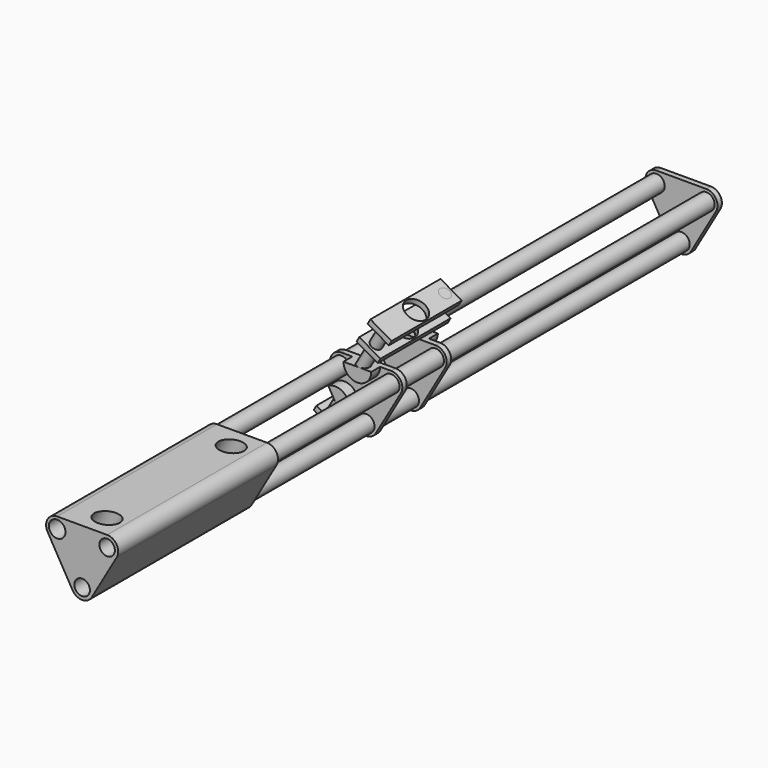
from build123d import *

# Parameters (mm, degrees)
F0_R      = 7.5
F0_R_2    = 7
F1_DEPTH  = 500
F3_DEPTH  = 5
F4_R      = 7.5
F5_DEPTH  = 180
F8_R      = 7
F9_DEPTH  = 25
F11_R     = 7
F12_DEPTH = 195.3
F15_DEPTH = 5
F18_DEPTH = 5
F20_DEPTH = 10
F22_DEPTH = 10
F24_R     = 5
F25_DEPTH = 50
F27_R     = 5
F28_DEPTH = 50
F29_W     = 22
F29_H     = 79
F30_DEPTH = 5
F31_R     = 10
F32_DEPTH = 28.9
F34_W     = 22
F34_H     = 79
F35_DEPTH = 5
F36_R     = 10
F37_DEPTH = 14.6
F39_DEPTH = 10
F41_DEPTH = 10
F44_R     = 5
F45_DEPTH = 25
F46_R     = 5
F47_DEPTH = 25.1
F48_W     = 22
F48_H     = 79
F48_R     = 5
F49_DEPTH = 5
F50_R     = 10
F51_DEPTH = 25
F52_R     = 5
F53_DEPTH = 25
F7_R      = 10
F56_DEPTH = 101


# Not quite as in the source:
# - a feature of the source that left no trace in its solid (it failed there, or was rolled back) is left out


with BuildPart() as f1:
    # F0 (on Front) → F1 (new body)
    with BuildSketch(Plane.XZ):
        with Locations((-22.5, 38.9711431703)):
            Circle(F0_R)
        with Locations((-22.5, 38.9711431703)):
            Circle(F0_R_2, mode=Mode.SUBTRACT)
    extrude(amount=F1_DEPTH)


with BuildPart() as f1b:
    # F0 (on Front) → F1, piece 2 (new body)
    with BuildSketch(Plane.XZ):
        with Locations((22.5, 38.9711431703)):
            Circle(F0_R)
        with Locations((22.5, 38.9711431703)):
            Circle(F0_R_2, mode=Mode.SUBTRACT)
    extrude(amount=F1_DEPTH)


with BuildPart() as f1c:
    # F0 (on Front) → F1, piece 3 (new body)
    with BuildSketch(Plane.XZ):
        Circle(F0_R)
        Circle(F0_R_2, mode=Mode.SUBTRACT)
    extrude(amount=F1_DEPTH)


with BuildPart() as f3:
    # F2 (on Front) → F3 (new body)
    with BuildSketch(Plane.XZ):
        with BuildLine():
            ThreePointArc((31.1602540378, 33.9711431703), (31.1602540378, 43.9711431703), (22.5, 48.9711431703))
            Line((22.5, 48.9711431703), (-22.5, 48.9711431703))
            ThreePointArc((-22.5, 48.9711431703), (-31.1602540378, 43.9711431703), (-31.1602540378, 33.9711431703))
            Line((-31.1602540378, 33.9711431703), (-8.6602540378, -5))
            ThreePointArc((-8.6602540378, -5), (0, -10), (8.6602540378, -5))
            Line((8.6602540378, -5), (31.1602540378, 33.9711431703))
        make_face()
    extrude(amount=F3_DEPTH)

    # F8 (on face) → F9 (cut)
    with BuildSketch(Plane(origin=(0, 0, 0), x_dir=(-1, 0, 0), z_dir=(0, 1, 0))):
        with Locations((-22.5, 38.9711431703)):
            Circle(F8_R)
        with Locations((22.5, 38.9711431703)):
            Circle(F8_R)
        Circle(F8_R)
    extrude(amount=-F9_DEPTH, mode=Mode.SUBTRACT)


with BuildPart() as f5:
    # F4 (on face) → F5 (new body)
    with BuildSketch(Plane.XZ.offset(500)):
        with BuildLine():
            Line((22.5, 48.9711431703), (-22.5, 48.9711431703))
            ThreePointArc((-22.5, 48.9711431703), (-31.1602540378, 43.9711431703), (-31.1602540378, 33.9711431703))
            Line((-31.1602540378, 33.9711431703), (-8.6602540378, -5))
            ThreePointArc((-8.6602540378, -5), (0, -10), (8.6602540378, -5))
            Line((8.6602540378, -5), (31.1602540378, 33.9711431703))
            ThreePointArc((31.1602540378, 33.9711431703), (31.1602540378, 43.9711431703), (22.5, 48.9711431703))
        make_face()
        with Locations((-22.5, 38.9711431703)):
            Circle(F4_R, mode=Mode.SUBTRACT)
    extrude(amount=F5_DEPTH)

    # F11 (on face) → F12 (cut)
    with BuildSketch(Plane.XZ.offset(680)):
        with Locations((22.5, 38.9711431703)):
            Circle(F11_R)
        Circle(F11_R)
        with Locations((-22.5, 38.9711431703)):
            Circle(F11_R)
    extrude(amount=-F12_DEPTH, mode=Mode.SUBTRACT)

    # F7 (on face) → F56 (cut)
    with BuildSketch(Plane(origin=(-4.3301270189, 0, -7.5), x_dir=(0.8660254038, 0, -0.5), z_dir=(0.5, 0, 0.8660254038))):
        with Locations((-18.9711431703, -660)):
            Circle(F7_R)
        with Locations((-18.9711431703, -520)):
            Circle(F7_R)
    extrude(amount=F56_DEPTH, mode=Mode.SUBTRACT)


with BuildPart() as f15:
    # F14 (on offset) → F15 (new body)
    with BuildSketch(Plane.XZ.offset(305)):
        with BuildLine():
            ThreePointArc((31.1602540378, 33.9711431703), (31.1602540378, 43.9711431703), (22.5, 48.9711431703))
            Line((22.5, 48.9711431703), (-22.5, 48.9711431703))
            ThreePointArc((-22.5, 48.9711431703), (-31.1602540378, 43.9711431703), (-31.1602540378, 33.9711431703))
            Line((-31.1602540378, 33.9711431703), (-8.6602540378, -5))
            ThreePointArc((-8.6602540378, -5), (0, -10), (8.6602540378, -5))
            Line((8.6602540378, -5), (31.1602540378, 33.9711431703))
        make_face()
    extrude(amount=F15_DEPTH)

    # F19 (on face) → F20 (join)
    with BuildSketch(Plane(origin=(0, -305, 0), x_dir=(-1, 0, 0), z_dir=(0, 1, 0))):
        with BuildLine():
            ThreePointArc((-12.5, 48.9711431703), (0, 36.4711431703), (12.5, 48.9711431703))
            Line((12.5, 48.9711431703), (-12.5, 48.9711431703))
        make_face()
    extrude(amount=F20_DEPTH)

    # F24 (on face) → F25 (join)
    with BuildSketch(Plane(origin=(18.0801270189, 0, 31.3156986041), x_dir=(0.8660254038, 0, -0.5), z_dir=(-0.5, 0, -0.8660254038))):
        with Locations((-23.3108891325, 300)):
            Circle(F24_R)
    extrude(amount=-F25_DEPTH)

    # F38 (on face) → F39 (join)
    with BuildSketch(Plane(origin=(0, -305, 0), x_dir=(-1, 0, 0), z_dir=(0, 1, 0))):
        with BuildLine():
            Line((13.6602540378, 3.6602540378), (26.1602540378, 25.3108891325))
            ThreePointArc((26.1602540378, 25.3108891325), (9.0849364905, 20.7355715851), (13.6602540378, 3.6602540378))
        make_face()
    extrude(amount=F39_DEPTH)

    # F44 (on face) → F45 (join)
    with BuildSketch(Plane(origin=(4.4198729811, 0, 7.6554445662), x_dir=(0.8660254038, 0, -0.5), z_dir=(-0.5, 0, -0.8660254038))):
        with Locations((-23.3108891325, 300)):
            Circle(F44_R)
    extrude(amount=F45_DEPTH)


with BuildPart() as f18:
    # F17 (on offset) → F18 (new body)
    with BuildSketch(Plane.XZ.offset(355)):
        with BuildLine():
            ThreePointArc((31.1602540378, 33.9711431703), (31.1602540378, 43.9711431703), (22.5, 48.9711431703))
            Line((22.5, 48.9711431703), (-22.5, 48.9711431703))
            ThreePointArc((-22.5, 48.9711431703), (-31.1602540378, 43.9711431703), (-31.1602540378, 33.9711431703))
            Line((-31.1602540378, 33.9711431703), (-8.6602540378, -5))
            ThreePointArc((-8.6602540378, -5), (0, -10), (8.6602540378, -5))
            Line((8.6602540378, -5), (31.1602540378, 33.9711431703))
        make_face()
    extrude(amount=F18_DEPTH)

    # F21 (on face) → F22 (join)
    with BuildSketch(Plane.XZ.offset(360)):
        with BuildLine():
            Line((12.5, 48.9711431703), (-12.5, 48.9711431703))
            ThreePointArc((-12.5, 48.9711431703), (0, 36.4711431703), (12.5, 48.9711431703))
        make_face()
    extrude(amount=F22_DEPTH)

    # F27 (on face) → F28 (join)
    with BuildSketch(Plane(origin=(18.0801270189, 0, 31.3156986041), x_dir=(0.8660254038, 0, -0.5), z_dir=(0.5, 0, 0.8660254038))):
        with Locations((-23.3108891325, -365)):
            Circle(F27_R)
    extrude(amount=F28_DEPTH)

    # F40 (on face) → F41 (join)
    with BuildSketch(Plane.XZ.offset(360)):
        with BuildLine():
            ThreePointArc((-13.6602540378, 3.6602540378), (-9.0849364905, 20.7355715851), (-26.1602540378, 25.3108891325))
            Line((-26.1602540378, 25.3108891325), (-13.6602540378, 3.6602540378))
        make_face()
    extrude(amount=F41_DEPTH)

    # F46 (on face) → F47 (join)
    with BuildSketch(Plane(origin=(4.4198729811, 0, 7.6554445662), x_dir=(0.8660254038, 0, -0.5), z_dir=(0.5, 0, 0.8660254038))):
        with Locations((-23.3108891325, -365)):
            Circle(F46_R)
    extrude(amount=-F47_DEPTH)

    # F48 (on face) → F49 (join)
    with BuildSketch(Plane(origin=(-8.0801270189, 0, -13.9951905284), x_dir=(0.8660254038, 0, -0.5), z_dir=(-0.5, 0, -0.8660254038))):
        with Locations((-23.3108891325, 332.5)):
            Rectangle(F48_W, F48_H)
        with Locations((-23.3108891325, 300)):
            Circle(F48_R, mode=Mode.SUBTRACT)
    extrude(amount=-F49_DEPTH)

    # F50 (on face) → F51 (cut)
    with BuildSketch(Plane(origin=(-8.0801270189, 0, -13.9951905284), x_dir=(0.8660254038, 0, -0.5), z_dir=(-0.5, 0, -0.8660254038))):
        with Locations((-23.3108891325, 332.5)):
            Circle(F50_R)
    extrude(amount=-F51_DEPTH, mode=Mode.SUBTRACT)


with BuildPart() as f30:
    # F29 (on face) → F30 (new body)
    with BuildSketch(Plane(origin=(43.0801270189, 0, 74.6169687933), x_dir=(0.8660254038, 0, -0.5), z_dir=(0.5, 0, 0.8660254038))):
        with Locations((-23.3108891325, -332.5)):
            Rectangle(F29_W, F29_H)
    extrude(amount=-F30_DEPTH)

    # F31 (on face) → F32 (cut)
    with BuildSketch(Plane(origin=(43.0801270189, 0, 74.6169687933), x_dir=(0.8660254038, 0, -0.5), z_dir=(0.5, 0, 0.8660254038))):
        with Locations((-23.3108891325, -332.5)):
            Circle(F31_R)
    extrude(amount=-F32_DEPTH, mode=Mode.SUBTRACT)


with BuildPart() as f35:
    # F34 (on offset) → F35 (new body)
    with BuildSketch(Plane(origin=(33.0801270189, 0, 57.2964607176), x_dir=(0.8660254038, 0, -0.5), z_dir=(-0.5, 0, -0.8660254038))):
        with Locations((-23.3108891325, 332.5)):
            Rectangle(F34_W, F34_H)
    extrude(amount=F35_DEPTH)

    # F36 (on face) → F37 (cut)
    with BuildSketch(Plane(origin=(33.0801270189, 0, 57.2964607176), x_dir=(0.8660254038, 0, -0.5), z_dir=(0.5, 0, 0.8660254038))):
        with Locations((-23.3108891325, -332.5)):
            Circle(F36_R)
    extrude(amount=-F37_DEPTH, mode=Mode.SUBTRACT)


with BuildPart() as f53_tool:
    # F52 (on face) → F53 (new body)
    with BuildSketch(Plane(origin=(43.0801270189, 0, 74.6169687933), x_dir=(0.8660254038, 0, -0.5), z_dir=(0.5, 0, 0.8660254038))):
        with Locations((-23.3108891325, -300)):
            Circle(F52_R)
    extrude(amount=-F53_DEPTH)


with BuildPart() as f30_1:
    add(f30.part)

    # F53: cut by f53_tool
    add(f53_tool.part, mode=Mode.SUBTRACT)


with BuildPart() as f35_1:
    add(f35.part)

    # F53: cut by f53_tool
    add(f53_tool.part, mode=Mode.SUBTRACT)


solid = Compound([f1.part, f1b.part, f1c.part, f3.part, f5.part, f15.part, f18.part, f30_1.part, f35_1.part])
